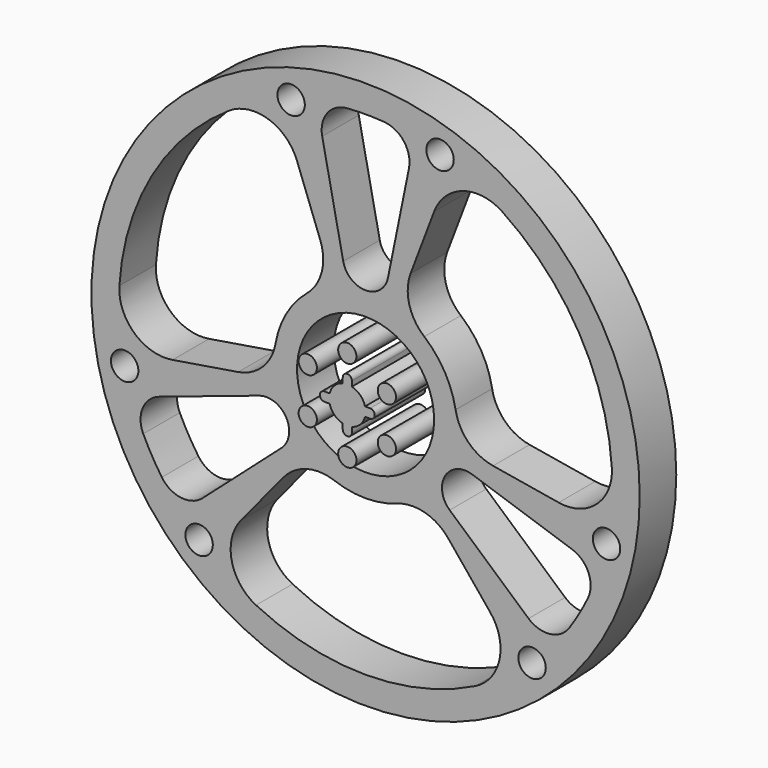
from build123d import *

# Parameters (mm, degrees)
F0_R     = 1524
F0_R_2   = 76.2
F0_R_3   = 381
F1_DEPTH = 127
F2_DEPTH = 254
F0_R_4   = 50.8


with BuildPart() as f1:
    # F0 (on Front) → F1 (new body, symmetric)
    with BuildSketch(Plane.XZ):
        Circle(F0_R)
        with Locations((-925.4829146604, -1012.3082211815)):
            Circle(F0_R_2, mode=Mode.SUBTRACT)
        with BuildLine():
            ThreePointArc((-1132.816748196, -773.3128571327), (-1187.8415809568, -685.798030436), (-1236.1189245676, -594.3875539796))
            ThreePointArc((-1236.1189245676, -594.3875539796), (-1239.1509183738, -469.0180629686), (-1147.1293372664, -383.8198771117))
            Line((-1147.1293372664, -383.8198771117), (-591.9889729048, -198.0313777959))
            ThreePointArc((-591.9889729048, -198.0313777959), (-441.7060552607, -254.9684820071), (-467.5385354179, -413.5858585473))
            Line((-467.5385354179, -413.5858585473), (-905.9649252706, -801.5300581884))
            ThreePointArc((-905.9649252706, -801.5300581884), (-1025.7596879891, -838.6237549571), (-1132.816748196, -773.3128571327))
        make_face(mode=Mode.SUBTRACT)
        with Locations((-1339.4265353536, -295.3355995993)):
            Circle(F0_R_2, mode=Mode.SUBTRACT)
        with BuildLine():
            ThreePointArc((-456.9716264903, -554.3509110508), (-327.7273635176, -470.8420273415), (-173.9859882065, -477.2765193342))
            ThreePointArc((-173.9859882065, -477.2765193342), (0, -508), (173.9859882065, -477.2765193342))
            ThreePointArc((173.9859882065, -477.2765193342), (328.2622454607, -469.9039091571), (458.2867111018, -553.2655146354))
            Line((458.2867111018, -553.2655146354), (692.2780797644, -839.8004645615))
            ThreePointArc((692.2780797644, -839.8004645615), (744.6718165916, -1054.4699417253), (609.0775800349, -1228.9471353557))
            ThreePointArc((609.0775800349, -1228.9471353557), (0, -1371.6), (-609.0775800349, -1228.9471353557))
            ThreePointArc((-609.0775800349, -1228.9471353557), (-744.6718165916, -1054.4699417253), (-692.2780797644, -839.8004645615))
            Line((-692.2780797644, -839.8004645615), (-456.9716264903, -554.3509110508))
        make_face(mode=Mode.SUBTRACT)
        with Locations((925.4813995717, -1012.3096063195)):
            Circle(F0_R_2, mode=Mode.SUBTRACT)
        with BuildLine():
            ThreePointArc((1236.116953448, -594.3916532039), (1187.8393067014, -685.8019695621), (1132.8141837234, -773.3166137844))
            ThreePointArc((1132.8141837234, -773.3166137844), (1025.7570165515, -838.6271429503), (905.9624326894, -801.5332089433))
            Line((905.9624326894, -801.5332089433), (467.49469037, -413.6618003978))
            ThreePointArc((467.49469037, -413.6618003978), (441.6622102128, -255.0444238576), (591.9451278569, -198.1073196465))
            Line((591.9451278569, -198.1073196465), (1147.1278549233, -383.8236111278))
            ThreePointArc((1147.1278549233, -383.8236111278), (1239.1493200045, -469.022070498), (1236.116953448, -594.3916532039))
        make_face(mode=Mode.SUBTRACT)
        with Locations((1339.4260933332, -295.3376042736)):
            Circle(F0_R_2, mode=Mode.SUBTRACT)
        with BuildLine():
            ThreePointArc((-500.3265844765, 87.9619739777), (-571.079845398, -49.3314890937), (-708.285346263, -120.2551767133))
            Line((-708.285346263, -120.2551767133), (-1073.4275763024, -179.6301712784))
            ThreePointArc((-1073.4275763024, -179.6301712784), (-1285.533665357, -117.669739788), (-1368.8382291435, 86.9969104921))
            ThreePointArc((-1368.8382291435, 86.9969104921), (-1187.8404438307, 685.8), (-759.7606491087, 1141.9502248636))
            ThreePointArc((-759.7606491087, 1141.9502248636), (-540.8618487654, 1172.1396815133), (-381.149496538, 1019.4306358399))
            Line((-381.149496538, 1019.4306358399), (-251.5961583359, 672.9244928747))
            ThreePointArc((-251.5961583359, 672.9244928747), (-243.8974750883, 519.2412359922), (-326.34059627, 389.3145453565))
            ThreePointArc((-326.34059627, 389.3145453565), (-439.9409051225, 254), (-500.3265844765, 87.9619739777))
        make_face(mode=Mode.SUBTRACT)
        with Locations((-413.9431786728, 1307.6458254551)):
            Circle(F0_R_2, mode=Mode.SUBTRACT)
        Circle(F0_R_3, mode=Mode.SUBTRACT)
        with BuildLine():
            ThreePointArc((326.34059627, 389.3145453565), (242.8175999373, 519.2353982508), (249.9986351612, 673.5206913487))
            Line((249.9986351612, 673.5206913487), (381.149496538, 1019.4306358399))
            ThreePointArc((381.149496538, 1019.4306358399), (540.8618487654, 1172.1396815133), (759.7606491087, 1141.9502248636))
            ThreePointArc((759.7606491087, 1141.9502248636), (1187.8404438307, 685.8), (1368.8382291435, 86.9969104921))
            ThreePointArc((1368.8382291435, 86.9969104921), (1285.533665357, -117.669739788), (1073.4275763024, -179.6301712784))
            Line((1073.4275763024, -179.6301712784), (708.5677848262, -118.5735818239))
            ThreePointArc((708.5677848262, -118.5735818239), (571.6248386059, -48.3992086508), (500.3265844765, 87.9619739777))
            ThreePointArc((500.3265844765, 87.9619739777), (439.9409051225, 254), (326.34059627, 389.3145453565))
        make_face(mode=Mode.SUBTRACT)
        with BuildLine():
            ThreePointArc((-103.300205252, 1367.7045103365), (0.0022742555, 1371.5999999981), (103.3047408442, 1367.704167764))
            ThreePointArc((103.3047408442, 1367.704167764), (213.3939018224, 1307.6452059188), (241.1669045771, 1185.353086055))
            Line((241.1669045771, 1185.353086055), (124.4942825347, 611.6931781937))
            ThreePointArc((124.4942825347, 611.6931781937), (0.0438450479, 510.0129058647), (-124.406592439, 611.6931781937))
            Line((-124.406592439, 611.6931781937), (-241.1629296527, 1185.3536693162))
            ThreePointArc((-241.1629296527, 1185.3536693162), (-213.3896320154, 1307.6458254551), (-103.300205252, 1367.7045103365))
        make_face(mode=Mode.SUBTRACT)
        with Locations((413.9451357819, 1307.6452059188)):
            Circle(F0_R_2, mode=Mode.SUBTRACT)
    extrude(amount=F1_DEPTH, both=True)


with BuildPart() as f2:
    # F0 (on Front) → F2 (new body, symmetric)
    with BuildSketch(Plane.XZ):
        with BuildLine():
            Line((-25.4040345891, 126.9999999359), (-25.4040345891, 98.372735179))
            ThreePointArc((-25.4040345891, 98.372735179), (-71.8435221849, 71.840575722), (-98.3737769937, 25.4))
            Line((-98.3737769937, 25.4), (-127, 25.4))
            ThreePointArc((-127, 25.4), (-152.3992151293, 0.199676781), (-127.3993412219, -25.3968605656))
            Line((-127.3993412219, -25.3968605656), (-98.3744028845, -25.3975758118))
            ThreePointArc((-98.3744028845, -25.3975758118), (-71.8444073469, -71.8396905128), (-25.4040345891, -98.372735179))
            Line((-25.4040345891, -98.372735179), (-25.4040345891, -126.9999999359))
            ThreePointArc((-25.4040345891, -126.9999999359), (-0.0040345891, -152.3999999359), (25.3959654109, -126.9999999359))
            Line((25.3959654109, -126.9999999359), (25.3959654109, -98.3748186318))
            ThreePointArc((25.3959654109, -98.3748186318), (71.8405757376, -71.8435221693), (98.3737769937, -25.4))
            Line((98.3737769937, -25.4), (127, -25.4))
            ThreePointArc((127, -25.4), (152.4, 0), (127, 25.4))
            Line((127, 25.4), (98.3737769937, 25.4))
            ThreePointArc((98.3737769937, 25.4), (71.8405757376, 71.8435221693), (25.3959654109, 98.3748186318))
            Line((25.3959654109, 98.3748186318), (25.3959654109, 126.9999999359))
            ThreePointArc((25.3959654109, 126.9999999359), (-0.0040345891, 152.3999999359), (-25.4040345891, 126.9999999359))
        make_face()
    extrude(amount=F2_DEPTH, both=True)


with BuildPart() as f2b:
    # F0 (on Front) → F2, piece 2 (new body, symmetric)
    with BuildSketch(Plane.XZ):
        with Locations((-0.0040345891, 253.999999968)):
            Circle(F0_R_4)
    extrude(amount=F2_DEPTH, both=True)


with BuildPart() as f2c:
    # F0 (on Front) → F2, piece 3 (new body, symmetric)
    with BuildSketch(Plane.XZ):
        with Locations((-219.9704525612, 127)):
            Circle(F0_R_4)
    extrude(amount=F2_DEPTH, both=True)


with BuildPart() as f2d:
    # F0 (on Front) → F2, piece 4 (new body, symmetric)
    with BuildSketch(Plane.XZ):
        with Locations((-219.968435239, -127.0034940406)):
            Circle(F0_R_4)
    extrude(amount=F2_DEPTH, both=True)


with BuildPart() as f2e:
    # F0 (on Front) → F2, piece 5 (new body, symmetric)
    with BuildSketch(Plane.XZ):
        with Locations((0, -254)):
            Circle(F0_R_4)
    extrude(amount=F2_DEPTH, both=True)


with BuildPart() as f2f:
    # F0 (on Front) → F2, piece 6 (new body, symmetric)
    with BuildSketch(Plane.XZ):
        with Locations((219.972469828, -126.9965059273)):
            Circle(F0_R_4)
    extrude(amount=F2_DEPTH, both=True)


with BuildPart() as f2g:
    # F0 (on Front) → F2, piece 7 (new body, symmetric)
    with BuildSketch(Plane.XZ):
        with Locations((219.9704525612, 127)):
            Circle(F0_R_4)
    extrude(amount=F2_DEPTH, both=True)


solid = Compound([f1.part, f2.part, f2b.part, f2c.part, f2d.part, f2e.part, f2f.part, f2g.part])
